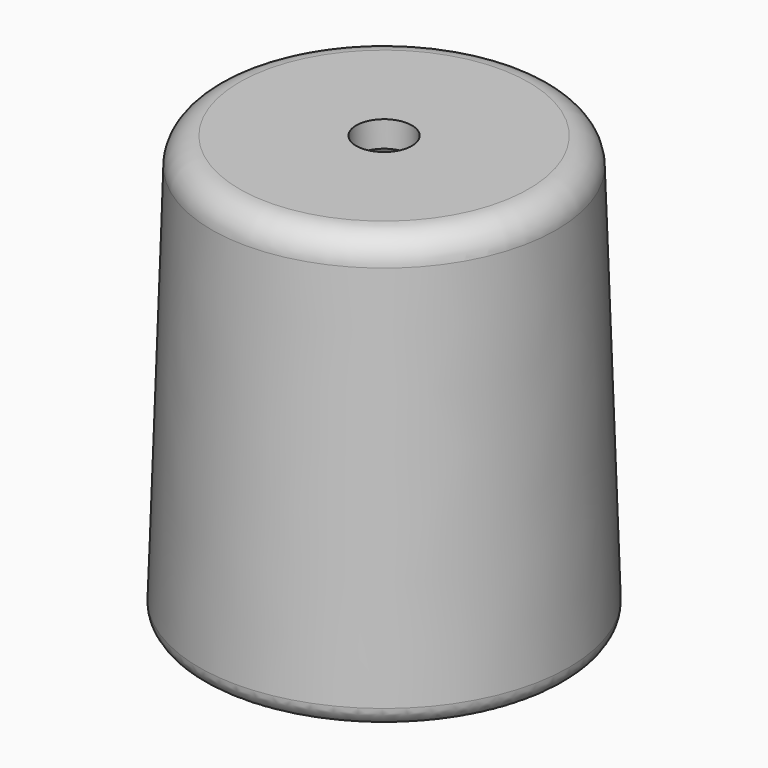
from build123d import *

# Parameters (mm, degrees)
F1_R     = 9
F1_R_2   = 6.9
F4_DEPTH = 3
F7_D     = 3
F7_DEPTH = 12
F7_TIP   = 0.9012909285
F8_R     = 1.5
F9_R     = 0.9999
F11_R    = 2


# Not quite as in the source:
# - a fillet or chamfer that OpenCascade refuses, or shapes differently, is made with other operations: its cross-section is extruded or revolved along the edge and cut away or added
# - a fillet or chamfer is up to 0.001 mm smaller than in the source, because OpenCascade refuses the exact size


with BuildPart() as f2:
    # F0 (on Front) → F2 (revolve)
    with BuildSketch(Plane.XZ):
        Polygon((0, 21.6), (0, 23), (-9.25, 23), (-10, 0), (-9.0005312399, -0.0325913726), (-8.5144306185, 14.6038573573), (-8.2820771734, 21.6), (-3.2820771734, 21.6), align=None)
        Polygon((-7.5149816695, 14.570664008), (-3.2820771734, 21.6), (-8.2820771734, 21.6), (-8.5144306185, 14.6038573573), align=None)
    revolve(axis=Axis((0, 0, 12.5640318729), (0, 0, -1)))

    # F0 (on Front) → F3 (revolve)
    with BuildSketch(Plane.XZ):
        Polygon((0, 21.6), (0, 23), (-9.25, 23), (-10, 0), (-9.0005312399, -0.0325913726), (-8.5144306185, 14.6038573573), (-8.2820771734, 21.6), (-3.2820771734, 21.6), align=None)
        Polygon((-7.5149816695, 14.570664008), (-3.2820771734, 21.6), (-8.2820771734, 21.6), (-8.5144306185, 14.6038573573), align=None)
    revolve(axis=Axis((0, 0, 12.5640318729), (0, 0, -1)))

    # F1 (on Top) → F4 (join)
    with BuildSketch(Plane.XY):
        Circle(F1_R)
        Circle(F1_R_2, mode=Mode.SUBTRACT)
    extrude(amount=F4_DEPTH)

    # F7
    with Locations(Plane.XY.offset(23)):
        with Locations((0, 0)):
            Hole(F7_D / 2, depth=F7_DEPTH)
            with Locations((0, 0, -(F7_DEPTH + F7_TIP / 2))):  # 118° drill point
                Cone(0, F7_D / 2, F7_TIP, mode=Mode.SUBTRACT)

    # F8
    f8_edges = [f2.edges().sort_by_distance(p)[0] for p in [
        (9.25, 0, 23),
    ]]
    fillet(f8_edges, radius=F8_R)

    # F9 (radius 1 in the source; OpenCascade refuses exactly that, so slightly less here)
    f9_edges = [f2.edges().sort_by_distance(p)[0] for p in [
        (10, 0, 0),
        (-6.9, 0, 0),
        (-6.9, 0, 3),
    ]]
    fillet(f9_edges, radius=F9_R)

    # F10: fillet of radius 2.5050114492 on 1 edges, made by hand

    # F10_s1 → F10_t2 (revolve, cut)
    with BuildSketch(Plane.XZ):
        with BuildLine():
            ThreePointArc((-6.7857760688, 15.781612939), (-7.5212900372, 15.0036690027), (-8.5144306185, 14.6038573573))
            Line((-8.5144306185, 14.6038573573), (-8.506084394, 14.5544572209))
            ThreePointArc((-8.506084394, 14.5544572209), (-8.0163691384, 14.5371880615), (-7.5166446639, 14.5205913868))
            Line((-7.5166446639, 14.5205913868), (-7.4720623541, 14.5448189832))
            Line((-7.4720623541, 14.5448189832), (-6.7428567534, 15.7557679142))
            Line((-6.7428567534, 15.7557679142), (-6.7857760688, 15.781612939))
        make_face()
    revolve(axis=Axis((0, 0, 14.570664008), (0, 0, -1)), mode=Mode.SUBTRACT)

    # F11
    f11_edges = [f2.edges().sort_by_distance(p)[0] for p in [
        (3.282077, 0, 21.6),
    ]]
    fillet(f11_edges, radius=F11_R)


solid = f2.part
